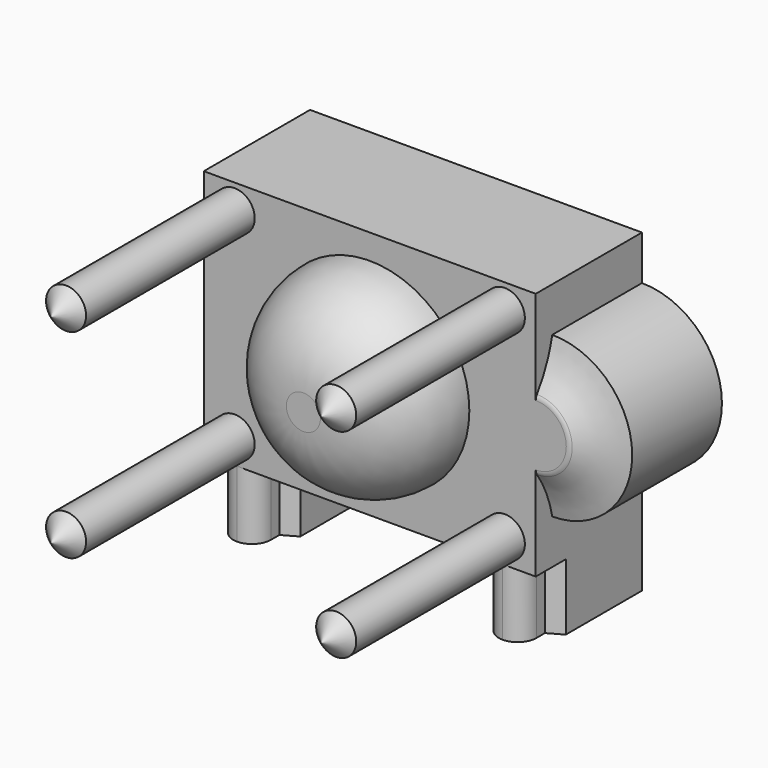
from build123d import *

# Parameters (mm, degrees)
F0_W         = 200
F0_H         = 150
F0_R         = 12.0683860383
F0_R_2       = 60
F1_DEPTH     = 80
F2_DEPTH     = 138
F3_C1_SIZE2  = 12
F3_C1_SIZE   = 11
F3_C2_SIZE2  = 12
F3_C2_SIZE   = 11
F3_C3_SIZE2  = 12
F3_C3_SIZE   = 11
F3_C4_SIZE2  = 12
F3_C4_SIZE   = 11
F4_DEPTH     = 50
F5_R         = 49.7327993849
F7_DEPTH     = 40
F8_DEPTH     = 20
F11_T2_ANGLE = 180


# Not quite as in the source:
# - a fillet or chamfer that OpenCascade refuses, or shapes differently, is made with other operations: its cross-section is extruded or revolved along the edge and cut away or added


with BuildPart() as f1:
    # F0 (on Front) → F1 (new body)
    with BuildSketch(Plane.XZ):
        Rectangle(F0_W, F0_H)
        with Locations((-81.3817187923, -60)):
            Circle(F0_R, mode=Mode.SUBTRACT)
        with Locations((81.3817187923, -60)):
            Circle(F0_R, mode=Mode.SUBTRACT)
        with Locations((-81.3817187923, 60)):
            Circle(F0_R, mode=Mode.SUBTRACT)
        Circle(F0_R_2, mode=Mode.SUBTRACT)
        with Locations((81.3817187923, 60)):
            Circle(F0_R, mode=Mode.SUBTRACT)
        Circle(F0_R_2)
        with Locations((81.3817187923, -60)):
            Circle(F0_R)
        with Locations((-81.3817187923, 60)):
            Circle(F0_R)
        with Locations((-81.3817187923, -60)):
            Circle(F0_R)
        with Locations((81.3817187923, 60)):
            Circle(F0_R)
    extrude(amount=-F1_DEPTH)

    # F0 (on Front) → F2 (join)
    with BuildSketch(Plane.XZ):
        with Locations((-81.3817187923, 60)):
            Circle(F0_R)
        with Locations((81.3817187923, 60)):
            Circle(F0_R)
        with Locations((81.3817187923, -60)):
            Circle(F0_R)
        with Locations((-81.3817187923, -60)):
            Circle(F0_R)
    extrude(amount=F2_DEPTH)

    # F3: chamfer of 12 x 11 on 4 edges, made by hand

    # F3_c1
    f3_c1_edges = [f1.edges().sort_by_distance(p)[0] for p in [
        (-93.4501048306, -138, -60),
    ]]
    f3_c1_side = f1.faces().sort_by_distance((-93.4501048306, -137.78, -60))[0]
    chamfer(f3_c1_edges, length=F3_C1_SIZE, length2=F3_C1_SIZE2, reference=f3_c1_side)

    # F3_c2
    f3_c2_edges = [f1.edges().sort_by_distance(p)[0] for p in [
        (69.313332754, -138, -60),
    ]]
    f3_c2_side = f1.faces().sort_by_distance((69.313332754, -137.78, -60))[0]
    chamfer(f3_c2_edges, length=F3_C2_SIZE, length2=F3_C2_SIZE2, reference=f3_c2_side)

    # F3_c3
    f3_c3_edges = [f1.edges().sort_by_distance(p)[0] for p in [
        (-93.4501048306, -138, 60),
    ]]
    f3_c3_side = f1.faces().sort_by_distance((-93.4501048306, -137.78, 60))[0]
    chamfer(f3_c3_edges, length=F3_C3_SIZE, length2=F3_C3_SIZE2, reference=f3_c3_side)

    # F3_c4
    f3_c4_edges = [f1.edges().sort_by_distance(p)[0] for p in [
        (69.313332754, -138, 60),
    ]]
    f3_c4_side = f1.faces().sort_by_distance((69.313332754, -137.78, 60))[0]
    chamfer(f3_c4_edges, length=F3_C4_SIZE, length2=F3_C4_SIZE2, reference=f3_c4_side)

    # F0 (on Front) → F4 (join)
    with BuildSketch(Plane.XZ):
        Circle(F0_R_2)
    extrude(amount=F4_DEPTH)

    # F5
    f5_edges = [f1.edges().sort_by_distance(p)[0] for p in [
        (-60, -50, 0),
    ]]
    fillet(f5_edges, radius=F5_R)

    # F6 (on face) → F7 (join)
    with BuildSketch(Plane(origin=(0, 0, -75), x_dir=(1, 0, 0), z_dir=(0, 0, -1))):
        with BuildLine():
            ThreePointArc((-68.6766029522, -11.3233970478), (-71.9931491676, -3.316546203), (-80.0000000175, 0))
            ThreePointArc((-80.0000000175, 0), (-88.0068508448, -3.3165462154), (-91.3233970478, -11.3233970478))
            Line((-91.3233970478, -11.3233970478), (-91.3233970478, -17.7343630829))
            Line((-91.3233970478, -17.7343630829), (-100, -22.6467940956))
            Line((-100, -22.6467940956), (-100, -80))
            Line((-100, -80), (-60, -80))
            Line((-60, -80), (-60, -22.6467940956))
            Line((-60, -22.6467940956), (-68.6766029522, -17.7343630829))
            Line((-68.6766029522, -17.7343630829), (-68.6766029522, -11.3233970478))
        make_face()
        with BuildLine():
            Line((68.6766029522, -17.7343630829), (60, -22.6467940956))
            Line((60, -22.6467940956), (60, -80))
            Line((60, -80), (100, -80))
            Line((100, -80), (100, -22.6467940956))
            Line((100, -22.6467940956), (91.3233970478, -17.7343630829))
            Line((91.3233970478, -17.7343630829), (91.3233970478, -11.3233970478))
            ThreePointArc((91.3233970478, -11.3233970478), (88.0068508386, -3.3165462092), (80, 0))
            ThreePointArc((80, 0), (71.9931491614, -3.3165462092), (68.6766029522, -11.3233970478))
            Line((68.6766029522, -11.3233970478), (68.6766029522, -17.7343630829))
        make_face()
    extrude(amount=F7_DEPTH)

    # F6 (on face) → F8 (cut)
    with BuildSketch(Plane(origin=(0, 0, -75), x_dir=(1, 0, 0), z_dir=(0, 0, -1))):
        with BuildLine():
            ThreePointArc((60, -80), (0, -20), (-60, -80))
            Line((-60, -80), (60, -80))
        make_face()
    extrude(amount=-F8_DEPTH, mode=Mode.SUBTRACT)

    # F9 (on face) → F10 (revolve)
    with BuildSketch(Plane.YZ.offset(100)):
        with BuildLine():
            Line((80, 0), (0, 0))
            Line((0, 0), (0, -20))
            ThreePointArc((0, -20), (7.7276234195, -33.4243037519), (12.4269118533, -48.1838695705))
            Line((12.4269118533, -48.1838695705), (80, -48.1838695705))
            Line((80, -48.1838695705), (80, 0))
        make_face()
    revolve(axis=Axis((100, 40, 0), (0, 1, 0)))

    # F11: fillet of radius 5 on 1 edges, made by hand

    # F11_s1 → F11_t2 (revolve, cut)
    with BuildSketch(Plane.YZ.offset(100)):
        with BuildLine():
            ThreePointArc((0, 18.4024363766), (0.2292975701, 19.8992323966), (0.8961593302, 21.2587437405))
            ThreePointArc((0.8961593302, 21.2587437405), (0.451433447, 20.6269841539), (0, 20))
            Line((0, 20), (0, 18.4024363766))
        make_face()
    revolve(axis=Axis((100, 0, 0), (0, 1, 0)), revolution_arc=F11_T2_ANGLE, mode=Mode.SUBTRACT)


solid = f1.part
